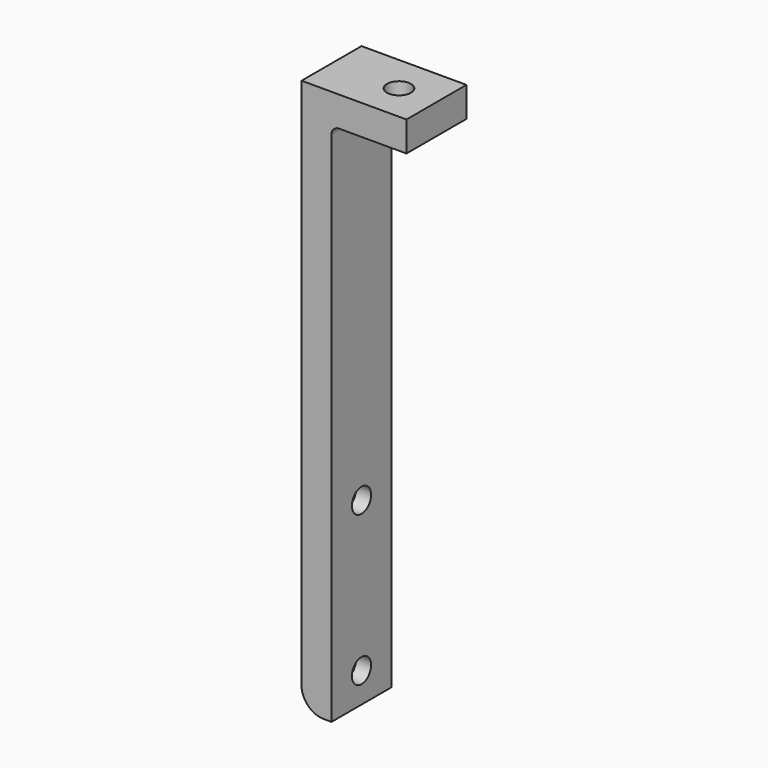
from build123d import *

# Parameters (mm, degrees)
F1_DEPTH             = 5
F4_D                 = 3.2
F4_CBORE_D           = 6.2
F4_CBORE_DEPTH       = 2
F4_ON_F3_D           = 3.2
F4_ON_F3_CBORE_D     = 6.2
F4_ON_F3_CBORE_DEPTH = 2
F5_R                 = 1
F6_T1_DEPTH          = 25


# Not quite as in the source:
# - a fillet or chamfer that OpenCascade refuses, or shapes differently, is made with other operations: its cross-section is extruded or revolved along the edge and cut away or added


with BuildPart() as f1:
    # F0 (on Front) → F1 (new body, symmetric)
    with BuildSketch(Plane.XZ):
        Polygon((0, 74), (0, 0), (4, 0), (4, 70), (14, 70), (14, 74), align=None)
    extrude(amount=F1_DEPTH, both=True)

    # F4 (through all)
    with Locations(Plane(origin=(0, 0, 0), x_dir=(0, -1, 0), z_dir=(-1, 0, 0))):
        with Locations((0, 24), (0, 4)):
            CounterBoreHole(F4_D / 2, F4_CBORE_D / 2, F4_CBORE_DEPTH)

    # F4 on F3 (through all)
    with Locations(Plane(origin=(0, 0, 70), x_dir=(1, 0, 0), z_dir=(0, 0, -1))):
        with Locations((9, 0)):
            CounterBoreHole(F4_ON_F3_D / 2, F4_ON_F3_CBORE_D / 2, F4_ON_F3_CBORE_DEPTH)

    # F5
    f5_edges = [f1.edges().sort_by_distance(p)[0] for p in [
        (4, 0, 70),
    ]]
    fillet(f5_edges, radius=F5_R)

    # F6: fillet of radius 3 on 1 edges, made by hand

    # F6_s2 → F6_t1 (cut)
    with BuildSketch(Plane.XZ.offset(-12.5)):
        with BuildLine():
            ThreePointArc((3, 0), (0.8786796564, 0.8786796564), (0, 3))
            Line((0, 3), (0, 0))
            Line((0, 0), (3, 0))
        make_face()
    extrude(amount=F6_T1_DEPTH, mode=Mode.SUBTRACT)


solid = f1.part
